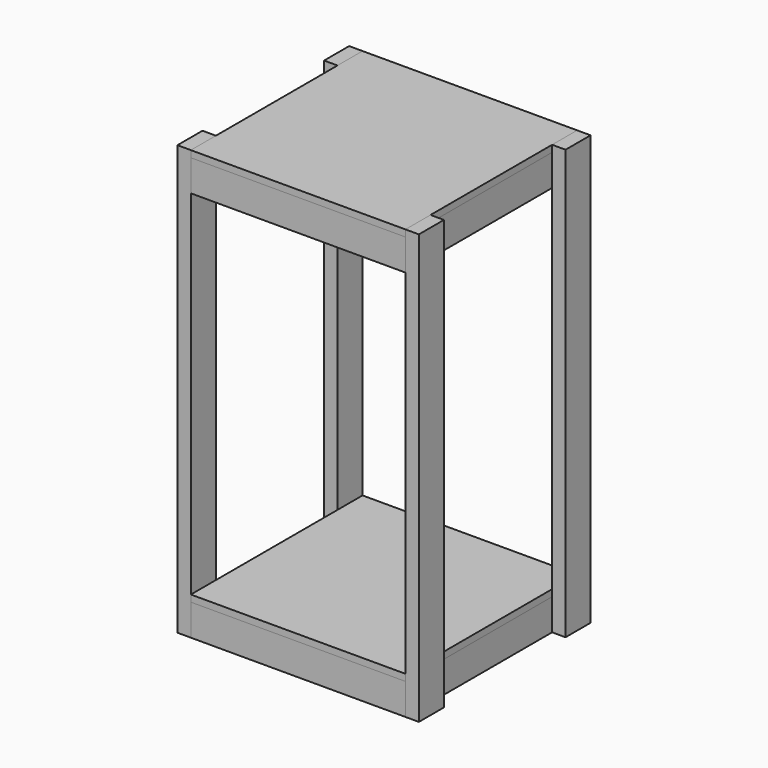
from build123d import *

# Parameters (mm, degrees)
F0_W          = 533.4
F0_H          = 533.4
F1_DEPTH      = 88.9
F2_W          = 38.1
F2_H          = 88.9
F3_DEPTH      = 1130.3
F3_DEPTH_BACK = 88.9
F4_W          = 609.6
F4_H          = 609.6
F5_DEPTH      = 19.05


# Not quite as in the source:
# - a feature of the source that left no trace in its solid (it failed there, or was rolled back) is left out
# - a pattern or mirror of a feature is missing from the dataset's text; its kind, count and spacing are read off the source's solid


with BuildPart() as f1:
    # F0 (on Top) → F1 (new body)
    with BuildSketch(Plane.XY):
        Polygon((-279.4, 304.8), (-304.8, 304.8), (-304.8, 215.9), (-304.8, -215.9), (-304.8, -304.8), (-279.4, -304.8), (304.8, -304.8), (304.8, -266.7), (304.8, -215.9), (304.8, 215.9), (304.8, 304.8), (-266.7, 304.8), align=None)
        Rectangle(F0_W, F0_H, mode=Mode.SUBTRACT)
    extrude(amount=F1_DEPTH)


with BuildPart() as f1_copies_1:
    # F1_copies: instance of F1
    add(f1.part.mirror(Plane.XY.offset(600.075)))


with BuildPart() as f3:
    # F2 (on face) → F3 (new body, two sides)
    with BuildSketch(Plane.XY.offset(88.9)) as f3_sk:
        with Locations((-323.85, 260.35)):
            Rectangle(F2_W, F2_H)
    extrude(amount=F3_DEPTH)
    extrude(f3_sk.sketch, amount=-F3_DEPTH_BACK)


with BuildPart() as f3b:
    # F2 (on face) → F3, piece 2 (new body, two sides)
    with BuildSketch(Plane.XY.offset(88.9)) as f3_2_sk:
        with Locations((323.85, 260.35)):
            Rectangle(F2_W, F2_H)
    extrude(amount=F3_DEPTH)
    extrude(f3_2_sk.sketch, amount=-F3_DEPTH_BACK)


with BuildPart() as f3c:
    # F2 (on face) → F3, piece 3 (new body, two sides)
    with BuildSketch(Plane.XY.offset(88.9)) as f3_3_sk:
        with Locations((323.85, -260.35)):
            Rectangle(F2_W, F2_H)
    extrude(amount=F3_DEPTH)
    extrude(f3_3_sk.sketch, amount=-F3_DEPTH_BACK)


with BuildPart() as f3d:
    # F2 (on face) → F3, piece 4 (new body, two sides)
    with BuildSketch(Plane.XY.offset(88.9)) as f3_4_sk:
        with Locations((-323.85, -260.35)):
            Rectangle(F2_W, F2_H)
    extrude(amount=F3_DEPTH)
    extrude(f3_4_sk.sketch, amount=-F3_DEPTH_BACK)


with BuildPart() as f5:
    # F4 (on face) → F5 (new body)
    with BuildSketch(Plane.XY.offset(88.9)):
        Rectangle(F4_W, F4_H)
    extrude(amount=F5_DEPTH)


with BuildPart() as f5_copies_1:
    # F5_copies: instance of F5
    add(f5.part.mirror(Plane.XY.offset(654.05)))


solid = Compound([f1.part, f1_copies_1.part, f3.part, f3b.part, f3c.part, f3d.part, f5.part, f5_copies_1.part])
